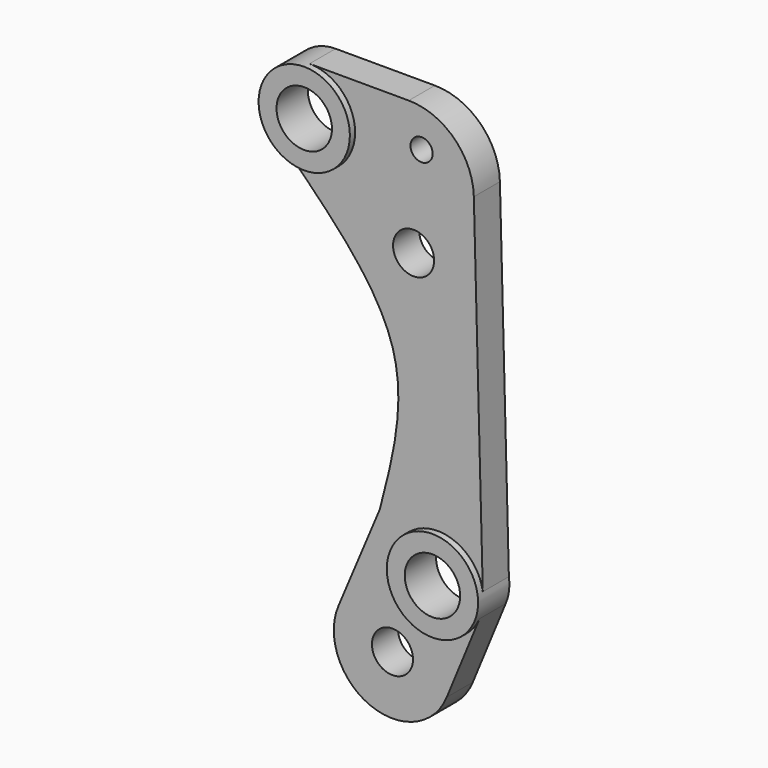
from build123d import *

# Parameters (mm, degrees)
F0_R     = 9
F0_R_2   = 3.4
F0_R_3   = 8.5
F0_R_4   = 6.3
F1_DEPTH = 10
F2_DEPTH = 12
F3_DEPTH = 10
F4_DEPTH = 10
F5_DEPTH = 10
F6_DEPTH = 12
F7_DEPTH = 10
F8_DEPTH = 10


# Not quite as in the source:
# - a feature names something its author has since deleted; it is built from what else it names


with BuildPart() as f1:
    # F0 (on Front) → F1 (new body)
    with BuildSketch(Plane.XZ):
        with BuildLine():
            ThreePointArc((57.9036016774, -19.5744080829), (31.1623185662, -12.2328702689), (58.8917768446, -11.9653941064))
            Line((58.8917768446, -11.9653941064), (56.1448434713, 93.81412645))
            ThreePointArc((56.1448434713, 93.81412645), (50.11852804, 107.6101149154), (36.1783402733, 113.2949139834))
            Line((36.1783402733, 113.2949139834), (5.7339191772, 113.3356434663))
            ThreePointArc((5.7339191772, 113.3356434663), (15.6213042052, 109.2285267967), (19.7151895633, 99.3356559948))
            ThreePointArc((19.7151895633, 99.3356559948), (13.3305472737, 87.5880465809), (0, 86.5553348621))
            add(Edge.make_bspline(
                [(27.2971690085, 0), (31.3022406236, 15.2863604375), (39.6477401648, 47.1390527935), (13.5652800367, 73.0692470789), (0, 86.5553348621)],
                knots=[0, 0, 0, 0, 0.4799079546, 1, 1, 1, 1], degree=3))
            Line((27.2971690085, 0), (14.5932951458, -30.2359827701))
            ThreePointArc((14.5932951458, -30.2359827701), (24.2784471497, -53.8293852547), (47.8350505361, -44.0550695737))
            Line((47.8350505361, -44.0550695737), (57.9036016774, -19.5744080829))
        make_face()
        with Locations((31.1880399704, -37.2083886825)):
            Circle(F0_R, mode=Mode.SUBTRACT)
        with Locations((37.6598948849, 72.601060337)):
            Circle(F0_R, mode=Mode.SUBTRACT)
        with Locations((40.1023646421, 101.2938035134)):
            Circle(F0_R_2, mode=Mode.SUBTRACT)
        with BuildLine():
            ThreePointArc((57.9036016774, -19.5744080829), (58.7572249195, -16.863419789), (59.0457295684, -14.0358952114))
            ThreePointArc((59.0457295684, -14.0358952114), (59.0071883365, -12.9977868034), (58.8917768446, -11.9653941064))
            ThreePointArc((58.8917768446, -11.9653941064), (31.1623185662, -12.2328702689), (57.9036016774, -19.5744080829))
        make_face()
        with Locations((45.0457295684, -14.0358952114)):
            Circle(F0_R_3, mode=Mode.SUBTRACT)
        with BuildLine():
            ThreePointArc((19.7151895633, 99.3356559948), (15.6213042052, 109.2285267967), (5.7339191772, 113.3356434663))
            ThreePointArc((5.7339191772, 113.3356434663), (-7.9745381996, 102.2667571151), (0, 86.5553348621))
            ThreePointArc((0, 86.5553348621), (13.3305472737, 87.5880465809), (19.7151895633, 99.3356559948))
        make_face()
        with Locations((5.7151895633, 99.3356559948)):
            Circle(F0_R_3, mode=Mode.SUBTRACT)
        with Locations((37.6598948849, 72.601060337)):
            Circle(F0_R)
        with Locations((37.6598948849, 72.601060337)):
            Circle(F0_R_4, mode=Mode.SUBTRACT)
        with Locations((31.1880399704, -37.2083886825)):
            Circle(F0_R)
        with Locations((31.1880399704, -37.2083886825)):
            Circle(F0_R_4, mode=Mode.SUBTRACT)
        with Locations((45.0457295684, -14.0358952114)):
            Circle(F0_R_3)
        with Locations((5.7151895633, 99.3356559948)):
            Circle(F0_R_3)
        with Locations((31.1880399704, -37.2083886825)):
            Circle(F0_R_4)
        with Locations((37.6598948849, 72.601060337)):
            Circle(F0_R_4)
        with Locations((40.1023646421, 101.2938035134)):
            Circle(F0_R_2)
    extrude(amount=F1_DEPTH)

    # F0 (on Front) → F2 (join)
    with BuildSketch(Plane.XZ):
        with BuildLine():
            ThreePointArc((19.7151895633, 99.3356559948), (15.6213042052, 109.2285267967), (5.7339191772, 113.3356434663))
            ThreePointArc((5.7339191772, 113.3356434663), (-7.9745381996, 102.2667571151), (0, 86.5553348621))
            ThreePointArc((0, 86.5553348621), (13.3305472737, 87.5880465809), (19.7151895633, 99.3356559948))
        make_face()
        with Locations((5.7151895633, 99.3356559948)):
            Circle(F0_R_3, mode=Mode.SUBTRACT)
    extrude(amount=F2_DEPTH)

    # F3 (cut): a face of the model
    f3_faces = [f1.faces().sort_by_distance(p)[0] for p in [
        (5.7151895633, -10, 99.3356559948),
    ]]
    extrude(f3_faces, amount=-F3_DEPTH, mode=Mode.SUBTRACT)

    # F0 (on Front) → F4 (cut)
    with BuildSketch(Plane.XZ):
        with Locations((40.1023646421, 101.2938035134)):
            Circle(F0_R_2)
    extrude(amount=F4_DEPTH, mode=Mode.SUBTRACT)

    # F0 (on Front) → F5 (cut)
    with BuildSketch(Plane.XZ):
        with Locations((37.6598948849, 72.601060337)):
            Circle(F0_R_4)
    extrude(amount=F5_DEPTH, mode=Mode.SUBTRACT)

    # F0 (on Front) → F6 (join)
    with BuildSketch(Plane.XZ):
        with BuildLine():
            ThreePointArc((57.9036016774, -19.5744080829), (58.7572249195, -16.863419789), (59.0457295684, -14.0358952114))
            ThreePointArc((59.0457295684, -14.0358952114), (59.0071883365, -12.9977868034), (58.8917768446, -11.9653941064))
            ThreePointArc((58.8917768446, -11.9653941064), (31.1623185662, -12.2328702689), (57.9036016774, -19.5744080829))
        make_face()
        with Locations((45.0457295684, -14.0358952114)):
            Circle(F0_R_3, mode=Mode.SUBTRACT)
    extrude(amount=F6_DEPTH)

    # F7 (cut): a face of the model
    f7_faces = [f1.faces().sort_by_distance(p)[0] for p in [
        (45.0457295684, -10, -14.0358952114),
    ]]
    extrude(f7_faces, amount=-F7_DEPTH, mode=Mode.SUBTRACT)

    # F0 (on Front) → F8 (cut)
    with BuildSketch(Plane.XZ):
        with Locations((31.1880399704, -37.2083886825)):
            Circle(F0_R_4)
    extrude(amount=F8_DEPTH, mode=Mode.SUBTRACT)


solid = f1.part
